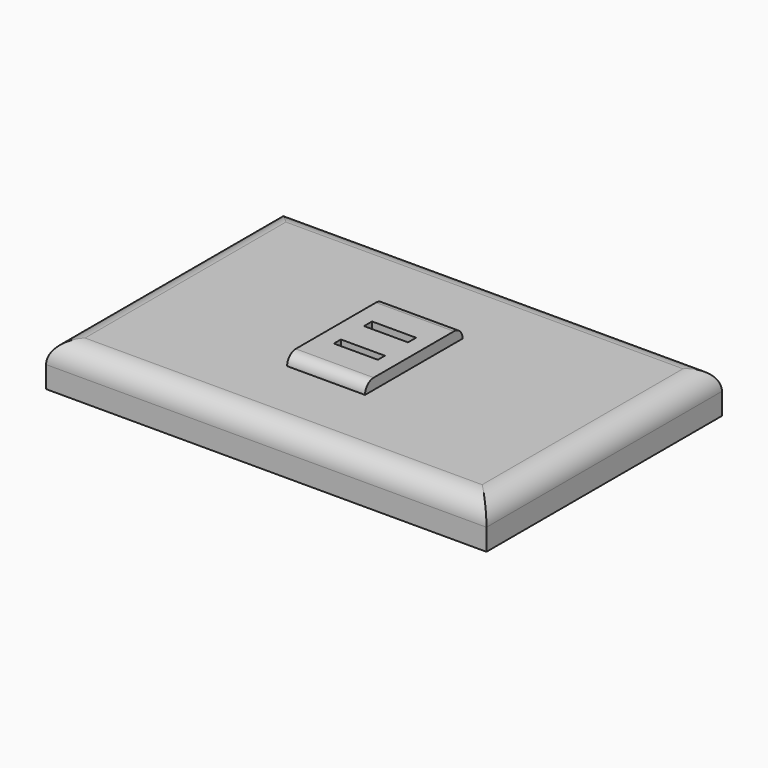
from build123d import *

# Parameters (mm, degrees)
F0_W     = 101.8128246069
F0_H     = 68.0426731706
F1_DEPTH = 10
F2_R     = 5
F3_W     = 18.016605638
F3_H     = 28.1872702762
F4_DEPTH = 2.5
F5_W     = 10.1706655696
F5_H     = 2.0341333002
F5_H_2   = 2.3247234058
F6_DEPTH = 25
F7_R     = 2.49999


# Not quite as in the source:
# - a fillet or chamfer is up to 0.001 mm smaller than in the source, because OpenCascade refuses the exact size


with BuildPart() as f1:
    # F0 (on Top) → F1 (new body)
    with BuildSketch(Plane.XY):
        with Locations((0.9539090097, -4.6469829977)):
            Rectangle(F0_W, F0_H)
    extrude(amount=F1_DEPTH)

    # F2
    f2_edges = [f1.edges().sort_by_distance(p)[0] for p in [
        (-49.952503, -4.646983, 10),
        (0.953909, 29.374354, 10),
        (0.953909, -38.66832, 10),
        (51.860321, -4.646983, 10),
    ]]
    fillet(f2_edges, radius=F2_R)

    # F3 (on face) → F4 (join)
    with BuildSketch(Plane.XY.offset(10)):
        with Locations((-0.5811811425, -5.3759221919)):
            Rectangle(F3_W, F3_H)
    extrude(amount=F4_DEPTH)

    # F5 (on face) → F6 (cut)
    with BuildSketch(Plane.XY.offset(12.5)):
        with Locations((-0.435885042, -10.0253690034)):
            Rectangle(F5_W, F5_H)
        with Locations((-0.435885042, -1.1623617029)):
            Rectangle(F5_W, F5_H_2)
    extrude(amount=-F6_DEPTH, mode=Mode.SUBTRACT)

    # F7 (radius 2.5 in the source; OpenCascade refuses exactly that, so slightly less here)
    f7_edges = [f1.edges().sort_by_distance(p)[0] for p in [
        (-0.581181, -19.469557, 12.5),
        (-0.581181, 8.717713, 12.5),
    ]]
    fillet(f7_edges, radius=F7_R)


solid = f1.part
